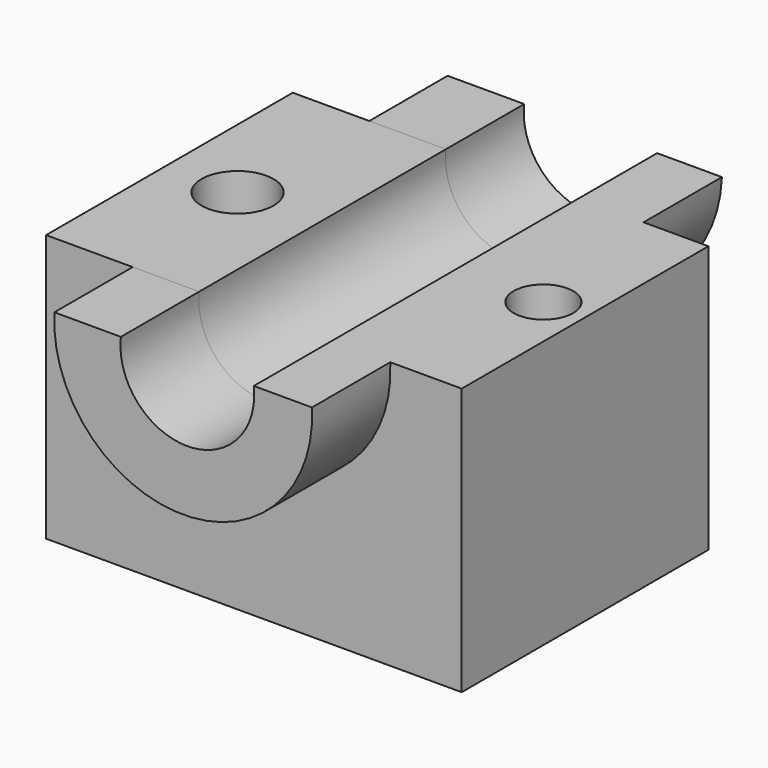
from build123d import *
from build123d import SkipClean  # not in build123d's __all__

# Parameters (mm, degrees)
F0_W     = 107.8271307051
F0_H     = 79.9957364798
F1_DEPTH = 69.342
F3_DEPTH = 171.704
F4_DEPTH = 25.4
F6_DEPTH = 25.4
F7_R     = 9.3550857854
F8_DEPTH = 220.218
F7_R_2   = 7.7300183475
F9_DEPTH = 194.31


# Not quite as in the source:
# - after a boolean that leaves OpenCascade's solid faulty, fix() repairs it


with BuildPart() as f1:
    # F0 (on Top) → F1 (new body)
    with BuildSketch(Plane.XY):
        with Locations((-0.6197858602, -6.3926763833)):
            Rectangle(F0_W, F0_H)
    extrude(amount=F1_DEPTH)

    # F2 (on face) → F3 (cut)
    with BuildSketch(Plane.XZ.offset(46.3905446231)):
        with BuildLine():
            Line((19.6710973978, 69.342), (-14.813689515, 69.342))
            ThreePointArc((-14.813689515, 69.342), (2.4287039414, 49.9755106866), (19.6710973978, 69.342))
        make_face()
    extrude(amount=-F3_DEPTH, mode=Mode.SUBTRACT)

    # F2 (on face) → F4 (join)
    with BuildSketch(Plane.XZ.offset(46.3905446231)):
        with BuildLine():
            Line((-14.813689515, 69.342), (-32.0560820401, 69.342))
            ThreePointArc((-32.0560820401, 69.342), (1.3510622084, 33.9996767093), (34.7582064569, 69.342))
            Line((34.7582064569, 69.342), (19.6710973978, 69.342))
            ThreePointArc((19.6710973978, 69.342), (2.4287039414, 49.9755106866), (-14.813689515, 69.342))
        make_face()
    with SkipClean():  # cleaning this boolean's faces spoils the solid; the shape is the same uncleaned
        extrude(amount=F4_DEPTH)

    # F5 (on face) → F6 (join)
    with BuildSketch(Plane(origin=(0, 33.6051918566, 0), x_dir=(-1, 0, 0), z_dir=(0, 1, 0))):
        with BuildLine():
            Line((-19.6710973978, 69.342), (-36.4824384451, 69.342))
            ThreePointArc((-36.4824384451, 69.342), (-0.9044590406, 35.2025825454), (34.6735203639, 69.342))
            Line((34.6735203639, 69.342), (14.813689515, 69.342))
            ThreePointArc((14.813689515, 69.342), (-2.4287039414, 49.9755106866), (-19.6710973978, 69.342))
        make_face()
    extrude(amount=F6_DEPTH)

    add(f1.part.fix(), mode=Mode.REPLACE)

    # F7 (on face) → F8 (cut)
    with BuildSketch(Plane.XY.offset(69.342)):
        with Locations((-35.963576287, -7.5180209242)):
            Circle(F7_R)
    extrude(amount=-F8_DEPTH, mode=Mode.SUBTRACT)

    # F7 (on face) → F9 (cut)
    with BuildSketch(Plane.XY.offset(69.342)):
        with Locations((42.4882248044, -6.3926763833)):
            Circle(F7_R_2)
    extrude(amount=-F9_DEPTH, mode=Mode.SUBTRACT)


solid = f1.part
